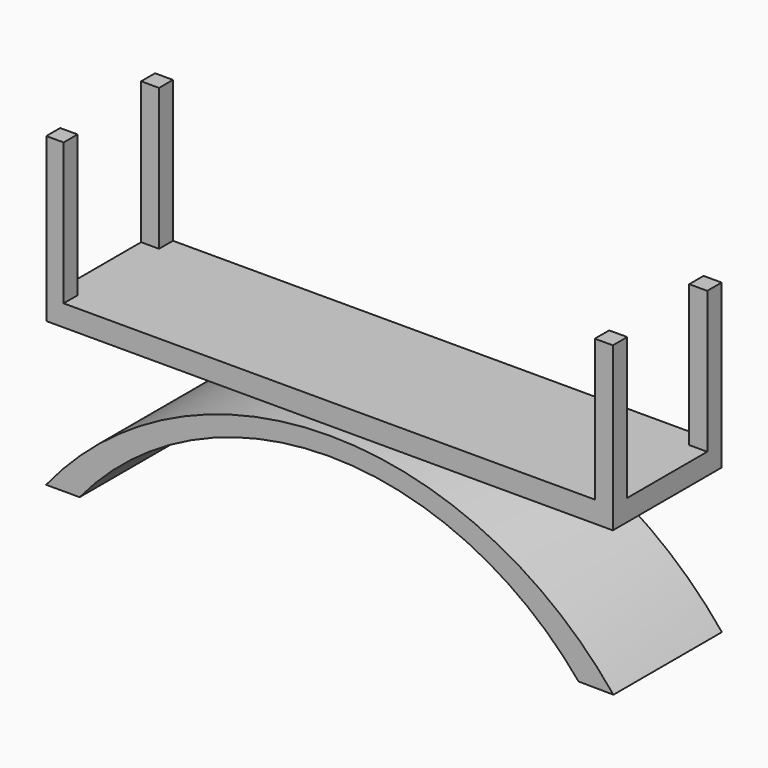
from build123d import *

# Parameters (mm, degrees)
F0_W     = 203.2
F0_H     = 7.62
F1_DEPTH = 48.76292
F2_W     = 6.4262472153
F2_H     = 6.2367809005
F2_W_2   = 6.2223918796
F2_H_2   = 6.2395843345
F2_W_3   = 6.4746759892
F2_H_3   = 6.4406376332
F2_H_4   = 6.4434433955
F3_DEPTH = 50.8
F5_DEPTH = 48.63821


# Not quite as in the source:
# - the program builds the solid bodies; features that only make, move or delete a surface that nothing else refers to are left out


with BuildPart() as f1:
    # F0 (on Front) → F1 (new body)
    with BuildSketch(Plane.XZ):
        Rectangle(F0_W, F0_H)
    extrude(amount=F1_DEPTH)

    # F2 (on face) → F3 (join)
    with BuildSketch(Plane.XY.offset(3.81)):
        with Locations((-98.3868763924, -3.1183904503)):
            Rectangle(F2_W, F2_H)
        with Locations((-98.4888040602, -45.6431278327)):
            Rectangle(F2_W_2, F2_H_2)
        with Locations((98.3626620054, -3.2203188166)):
            Rectangle(F2_W_3, F2_H_3)
        with Locations((98.3626620054, -45.5411983022)):
            Rectangle(F2_W_3, F2_H_4)
    extrude(amount=F3_DEPTH)


with BuildPart() as f5:
    # F4 (on Front) → F5 (new body)
    with BuildSketch(Plane.XZ):
        with BuildLine():
            Line((89.2202242982, -55.6125417352), (101.708002892, -55.7293946085))
            ThreePointArc((101.708002892, -55.7293946085), (-0.0027350897, -7.001500307), (-101.7693728209, -55.6125417352))
            Line((-101.7693728209, -55.6125417352), (-89.7364146949, -55.6125417352))
            ThreePointArc((-89.7364146949, -55.6125417352), (-0.2580951983, -13.5554328116), (89.2202242982, -55.6125417352))
        make_face()
    extrude(amount=F5_DEPTH)


solid = Compound([f1.part, f5.part])
